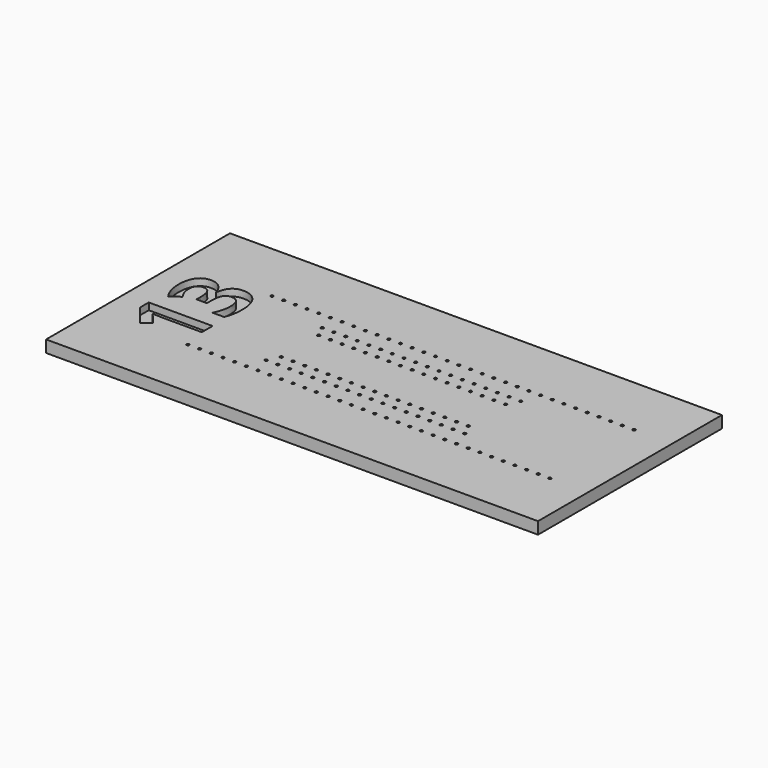
from build123d import *

# Parameters (mm, degrees)
F0_W         = 107
F0_H         = 50
F1_DEPTH     = 2.6
F2_TEXT_SIZE = 19.4444444444
F3_DEPTH     = 1.5
F4_R         = 0.3
F5_DEPTH     = 2.6


# Not quite as in the source:
# - Text() gives the source's letters only with a copy of the font that has no kerning and outlines rounded to 1/6400 em; it was checked with that copy


with BuildPart() as f1:
    # F0 (on Top) → F1 (new body)
    with BuildSketch(Plane.XY):
        with Locations((10.3412768841, 3.3350909071)):
            Rectangle(F0_W, F0_H)
    extrude(amount=F1_DEPTH)

    # F2 (on face) → F3 (cut)
    with BuildSketch(Plane.XY.offset(2.6)):
        with Locations(Location((-24.1587231159, -8.1723743707), (0, 0, 90))):
            Text('13', F2_TEXT_SIZE, font='Open Sans', font_style=FontStyle.BOLD, text_align=(TextAlign.LEFT, TextAlign.BOTTOM))
    extrude(amount=-F3_DEPTH, mode=Mode.SUBTRACT)

    # F4 (on face) → F5 (cut, through all)
    with BuildSketch(Plane.XY.offset(2.6)):
        with Locations((-23.1587231159, 14.7650909071)):
            Circle(F4_R)
        with Locations((-20.6187231159, 14.7650909071)):
            Circle(F4_R)
        with Locations((-18.0787231159, 14.7650909071)):
            Circle(F4_R)
        with Locations((-15.5387231159, 14.7650909071)):
            Circle(F4_R)
        with Locations((-12.9987231159, 14.7650909071)):
            Circle(F4_R)
        with Locations((-10.4587231159, 14.7650909071)):
            Circle(F4_R)
        with Locations((-7.9187231159, 14.7650909071)):
            Circle(F4_R)
        with Locations((-5.3787231159, 14.7650909071)):
            Circle(F4_R)
        with Locations((-2.8387231159, 14.7650909071)):
            Circle(F4_R)
        with Locations((-0.2987231159, 14.7650909071)):
            Circle(F4_R)
        with Locations((2.2412768841, 14.7650909071)):
            Circle(F4_R)
        with Locations((4.7812768841, 14.7650909071)):
            Circle(F4_R)
        with Locations((7.3212768841, 14.7650909071)):
            Circle(F4_R)
        with Locations((9.8612768841, 14.7650909071)):
            Circle(F4_R)
        with Locations((12.4012768841, 14.7650909071)):
            Circle(F4_R)
        with Locations((14.9412768841, 14.7650909071)):
            Circle(F4_R)
        with Locations((17.4812768841, 14.7650909071)):
            Circle(F4_R)
        with Locations((20.0212768841, 14.7650909071)):
            Circle(F4_R)
        with Locations((22.5612768841, 14.7650909071)):
            Circle(F4_R)
        with Locations((25.1012768841, 14.7650909071)):
            Circle(F4_R)
        with Locations((27.6412768841, 14.7650909071)):
            Circle(F4_R)
        with Locations((30.1812768841, 14.7650909071)):
            Circle(F4_R)
        with Locations((32.7212768841, 14.7650909071)):
            Circle(F4_R)
        with Locations((35.2612768841, 14.7650909071)):
            Circle(F4_R)
        with Locations((37.8012768841, 14.7650909071)):
            Circle(F4_R)
        with Locations((40.3412768841, 14.7650909071)):
            Circle(F4_R)
        with Locations((42.8812768841, 14.7650909071)):
            Circle(F4_R)
        with Locations((45.4212768841, 14.7650909071)):
            Circle(F4_R)
        with Locations((47.9612768841, 14.7650909071)):
            Circle(F4_R)
        with Locations((50.5012768841, 14.7650909071)):
            Circle(F4_R)
        with Locations((53.0412768841, 14.7650909071)):
            Circle(F4_R)
        with Locations((55.5812768841, 14.7650909071)):
            Circle(F4_R)
        with Locations((-23.1587231159, -8.0949090929)):
            Circle(F4_R)
        with Locations((-20.6187231159, -8.0949090929)):
            Circle(F4_R)
        with Locations((-18.0787231159, -8.0949090929)):
            Circle(F4_R)
        with Locations((-15.5387231159, -8.0949090929)):
            Circle(F4_R)
        with Locations((-12.9987231159, -8.0949090929)):
            Circle(F4_R)
        with Locations((-10.4587231159, -8.0949090929)):
            Circle(F4_R)
        with Locations((-7.9187231159, -8.0949090929)):
            Circle(F4_R)
        with Locations((-5.3787231159, -8.0949090929)):
            Circle(F4_R)
        with Locations((-2.8387231159, -8.0949090929)):
            Circle(F4_R)
        with Locations((-0.2987231159, -8.0949090929)):
            Circle(F4_R)
        with Locations((2.2412768841, -8.0949090929)):
            Circle(F4_R)
        with Locations((4.7812768841, -8.0949090929)):
            Circle(F4_R)
        with Locations((7.3212768841, -8.0949090929)):
            Circle(F4_R)
        with Locations((9.8612768841, -8.0949090929)):
            Circle(F4_R)
        with Locations((12.4012768841, -8.0949090929)):
            Circle(F4_R)
        with Locations((14.9412768841, -8.0949090929)):
            Circle(F4_R)
        with Locations((17.4812768841, -8.0949090929)):
            Circle(F4_R)
        with Locations((20.0212768841, -8.0949090929)):
            Circle(F4_R)
        with Locations((22.5612768841, -8.0949090929)):
            Circle(F4_R)
        with Locations((25.1012768841, -8.0949090929)):
            Circle(F4_R)
        with Locations((27.6412768841, -8.0949090929)):
            Circle(F4_R)
        with Locations((30.1812768841, -8.0949090929)):
            Circle(F4_R)
        with Locations((32.7212768841, -8.0949090929)):
            Circle(F4_R)
        with Locations((35.2612768841, -8.0949090929)):
            Circle(F4_R)
        with Locations((37.8012768841, -8.0949090929)):
            Circle(F4_R)
        with Locations((40.3412768841, -8.0949090929)):
            Circle(F4_R)
        with Locations((42.8812768841, -8.0949090929)):
            Circle(F4_R)
        with Locations((45.4212768841, -8.0949090929)):
            Circle(F4_R)
        with Locations((47.9612768841, -8.0949090929)):
            Circle(F4_R)
        with Locations((50.5012768841, -8.0949090929)):
            Circle(F4_R)
        with Locations((53.0412768841, -8.0949090929)):
            Circle(F4_R)
        with Locations((55.5812768841, -8.0949090929)):
            Circle(F4_R)
        with Locations((-9.1887231159, 10.9550909071)):
            Circle(F4_R)
        with Locations((-6.6487231159, 10.9550909071)):
            Circle(F4_R)
        with Locations((-4.1087231159, 10.9550909071)):
            Circle(F4_R)
        with Locations((-1.5687231159, 10.9550909071)):
            Circle(F4_R)
        with Locations((0.9712768841, 10.9550909071)):
            Circle(F4_R)
        with Locations((3.5112768841, 10.9550909071)):
            Circle(F4_R)
        with Locations((6.0512768841, 10.9550909071)):
            Circle(F4_R)
        with Locations((8.5912768841, 10.9550909071)):
            Circle(F4_R)
        with Locations((11.1312768841, 10.9550909071)):
            Circle(F4_R)
        with Locations((13.6712768841, 10.9550909071)):
            Circle(F4_R)
        with Locations((16.2112768841, 10.9550909071)):
            Circle(F4_R)
        with Locations((18.7512768841, 10.9550909071)):
            Circle(F4_R)
        with Locations((21.2912768841, 10.9550909071)):
            Circle(F4_R)
        with Locations((23.8312768841, 10.9550909071)):
            Circle(F4_R)
        with Locations((26.3712768841, 10.9550909071)):
            Circle(F4_R)
        with Locations((28.9112768841, 10.9550909071)):
            Circle(F4_R)
        with Locations((31.4512768841, 10.9550909071)):
            Circle(F4_R)
        with Locations((33.9912768841, 10.9550909071)):
            Circle(F4_R)
        with Locations((-7.9187231159, 8.4150909071)):
            Circle(F4_R)
        with Locations((-5.3787231159, 8.4150909071)):
            Circle(F4_R)
        with Locations((-2.8387231159, 8.4150909071)):
            Circle(F4_R)
        with Locations((-0.2987231159, 8.4150909071)):
            Circle(F4_R)
        with Locations((2.2412768841, 8.4150909071)):
            Circle(F4_R)
        with Locations((4.7812768841, 8.4150909071)):
            Circle(F4_R)
        with Locations((7.3212768841, 8.4150909071)):
            Circle(F4_R)
        with Locations((9.8612768841, 8.4150909071)):
            Circle(F4_R)
        with Locations((12.4012768841, 8.4150909071)):
            Circle(F4_R)
        with Locations((14.9412768841, 8.4150909071)):
            Circle(F4_R)
        with Locations((17.4812768841, 8.4150909071)):
            Circle(F4_R)
        with Locations((20.0212768841, 8.4150909071)):
            Circle(F4_R)
        with Locations((22.5612768841, 8.4150909071)):
            Circle(F4_R)
        with Locations((25.1012768841, 8.4150909071)):
            Circle(F4_R)
        with Locations((27.6412768841, 8.4150909071)):
            Circle(F4_R)
        with Locations((30.1812768841, 8.4150909071)):
            Circle(F4_R)
        with Locations((32.7212768841, 8.4150909071)):
            Circle(F4_R)
        with Locations((-9.1887231159, -4.2849090929)):
            Circle(F4_R)
        with Locations((-6.6487231159, -4.2849090929)):
            Circle(F4_R)
        with Locations((-4.1087231159, -4.2849090929)):
            Circle(F4_R)
        with Locations((-1.5687231159, -4.2849090929)):
            Circle(F4_R)
        with Locations((0.9712768841, -4.2849090929)):
            Circle(F4_R)
        with Locations((3.5112768841, -4.2849090929)):
            Circle(F4_R)
        with Locations((6.0512768841, -4.2849090929)):
            Circle(F4_R)
        with Locations((8.5912768841, -4.2849090929)):
            Circle(F4_R)
        with Locations((11.1312768841, -4.2849090929)):
            Circle(F4_R)
        with Locations((13.6712768841, -4.2849090929)):
            Circle(F4_R)
        with Locations((16.2112768841, -4.2849090929)):
            Circle(F4_R)
        with Locations((18.7512768841, -4.2849090929)):
            Circle(F4_R)
        with Locations((21.2912768841, -4.2849090929)):
            Circle(F4_R)
        with Locations((23.8312768841, -4.2849090929)):
            Circle(F4_R)
        with Locations((26.3712768841, -4.2849090929)):
            Circle(F4_R)
        with Locations((28.9112768841, -4.2849090929)):
            Circle(F4_R)
        with Locations((31.4512768841, -4.2849090929)):
            Circle(F4_R)
        with Locations((33.9912768841, -4.2849090929)):
            Circle(F4_R)
        with Locations((-7.9187231159, -1.7449090929)):
            Circle(F4_R)
        with Locations((-5.3787231159, -1.7449090929)):
            Circle(F4_R)
        with Locations((-2.8387231159, -1.7449090929)):
            Circle(F4_R)
        with Locations((-0.2987231159, -1.7449090929)):
            Circle(F4_R)
        with Locations((2.2412768841, -1.7449090929)):
            Circle(F4_R)
        with Locations((4.7812768841, -1.7449090929)):
            Circle(F4_R)
        with Locations((7.3212768841, -1.7449090929)):
            Circle(F4_R)
        with Locations((9.8612768841, -1.7449090929)):
            Circle(F4_R)
        with Locations((12.4012768841, -1.7449090929)):
            Circle(F4_R)
        with Locations((14.9412768841, -1.7449090929)):
            Circle(F4_R)
        with Locations((17.4812768841, -1.7449090929)):
            Circle(F4_R)
        with Locations((20.0212768841, -1.7449090929)):
            Circle(F4_R)
        with Locations((22.5612768841, -1.7449090929)):
            Circle(F4_R)
        with Locations((25.1012768841, -1.7449090929)):
            Circle(F4_R)
        with Locations((27.6412768841, -1.7449090929)):
            Circle(F4_R)
        with Locations((30.1812768841, -1.7449090929)):
            Circle(F4_R)
        with Locations((32.7212768841, -1.7449090929)):
            Circle(F4_R)
    extrude(amount=-F5_DEPTH, mode=Mode.SUBTRACT)


solid = f1.part
